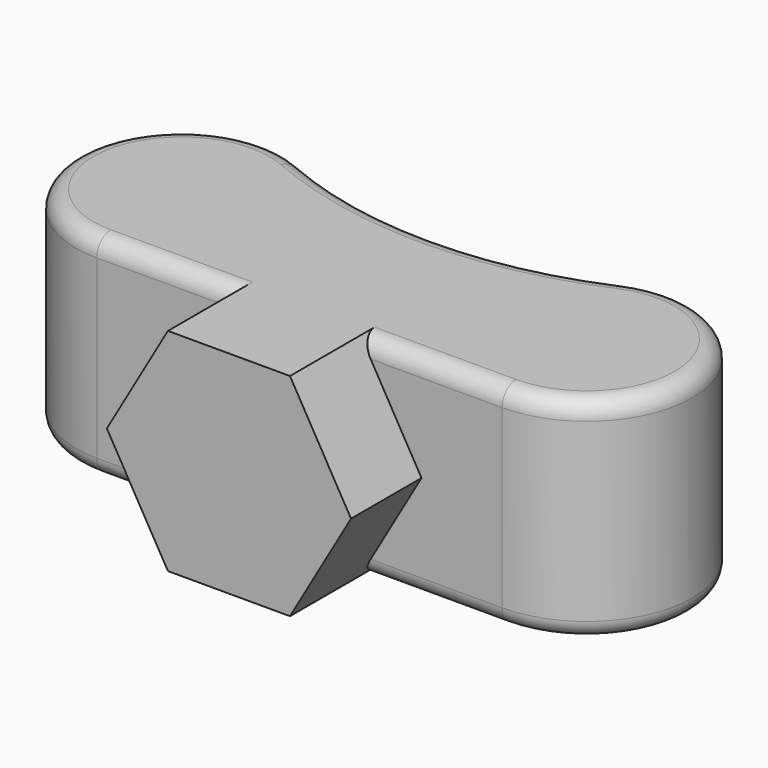
from build123d import *

# Parameters (mm, degrees)
F1_DEPTH = 5
F3_DEPTH = 12
F4_R     = 1


# Not quite as in the source:
# - a feature names something its author has since deleted; it is built from what else it names


with BuildPart() as f1:
    # F0 (on Front) → F1 (new body)
    with BuildSketch(Plane.XZ):
        Polygon((3.4641016151, 0), (6.9282032303, 6), (3.4641016151, 12), (-3.4641016151, 12), (-6.9282032303, 6), (-3.4641016151, 0), align=None)
    extrude(amount=F1_DEPTH)

    # F2 (on Top) → F3 (join)
    with BuildSketch(Plane.XY):
        with BuildLine():
            ThreePointArc((-9.1206896552, 11.5080742808), (-17.3757316857, 7.2148156887), (-11.5, 0))
            Line((-11.5, 0), (11.5, 0))
            ThreePointArc((11.5, 0), (17.3757316857, 7.2148156887), (9.1206896552, 11.5080742808))
            ThreePointArc((9.1206896552, 11.5080742808), (0, 9.6223590239), (-9.1206896552, 11.5080742808))
        make_face()
    extrude(amount=F3_DEPTH)

    # F4
    f4_edges = [f1.edges().sort_by_distance(p)[0] for p in [
        (7.482051, 0, 12),
        (7.482051, 0, 0),
    ]]
    fillet(f4_edges, radius=F4_R)


solid = f1.part
